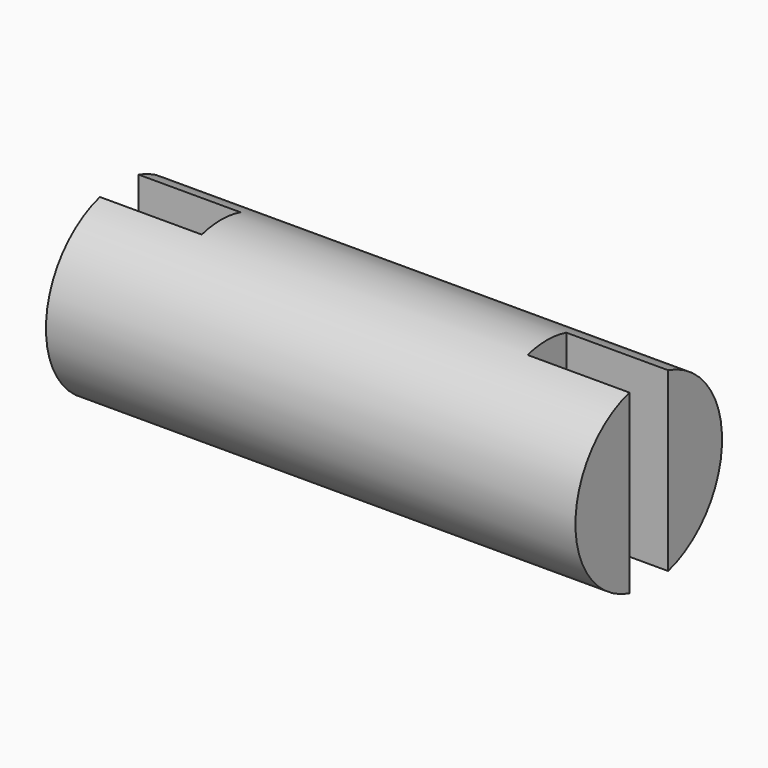
from build123d import *

# Parameters (mm, degrees)
F0_W     = 13
F0_H     = 2.25
F3_DEPTH = 2.5


# Not quite as in the source:
# - a pattern or mirror of a feature is missing from the dataset's text; its kind, count and spacing are read off the source's solid


with BuildPart() as f1:
    # F0 (on Front) → F1 (revolve)
    with BuildSketch(Plane.XZ):
        with Locations((6.5, 1.125)):
            Rectangle(F0_W, F0_H)
    revolve(axis=Axis((6.5, 0, 0), (1, 0, 0)))

    # F2 (on face) → F3 (cut)
    with BuildSketch(Plane.YZ.offset(13)):
        with BuildLine():
            Line((0.5940446135, -2.170163818), (0.5940446135, 2.170163818))
            ThreePointArc((0.5940446135, 2.170163818), (0, 2.25), (-0.5940446135, 2.170163818))
            Line((-0.5940446135, 2.170163818), (-0.5940446135, -2.170163818))
            ThreePointArc((-0.5940446135, -2.170163818), (0, -2.25), (0.5940446135, -2.170163818))
        make_face()
    f3 = extrude(amount=-F3_DEPTH, mode=Mode.SUBTRACT)

    # F3_copies: F3 across plane
    add(f3.mirror(Plane(origin=(6.5, 0, 0), x_dir=(0, 0, -1), z_dir=(-1, 0, 0))), mode=Mode.SUBTRACT)


solid = f1.part
